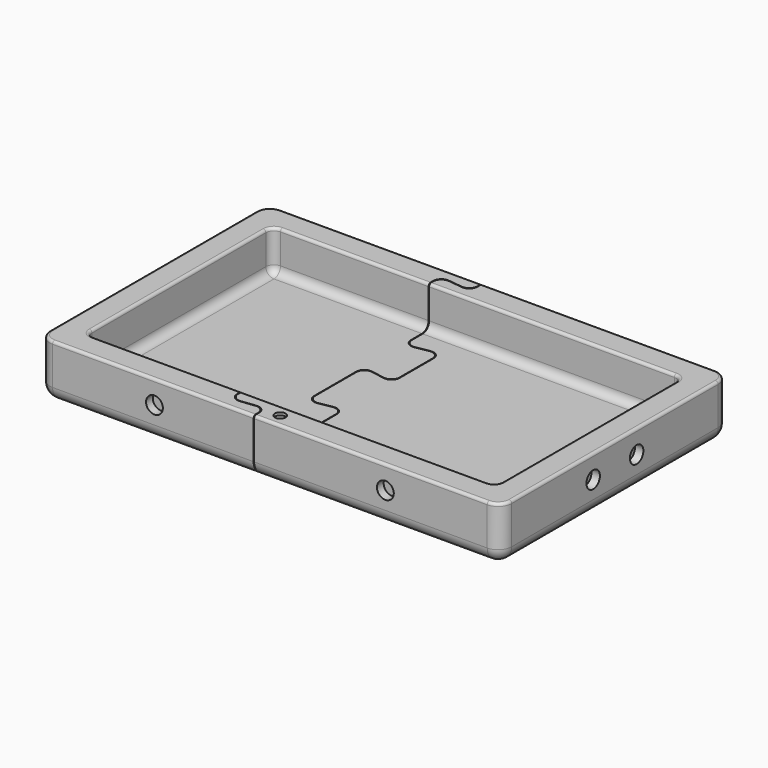
from build123d import *

# Parameters (mm, degrees)
F0_W      = 170
F0_H      = 105
F0_R      = 2
F3_DEPTH  = 20
F4_DEPTH  = 15
F5_R      = 5
F6_R      = 3
F7_R      = 1
F8_R      = 3.1
F9_DEPTH  = 3.1
F10_R     = 3.1
F11_DEPTH = 3.1
F12_R     = 3.1
F13_DEPTH = 3.1
F14_R     = 3.1
F15_DEPTH = 3.1
F16_DEPTH = 1
F17_ANGLE = 180
F19_DEPTH = 25
F20_DEPTH = 25


# Not quite as in the source:
# - a feature names something its author has since deleted; it is built from what else it names


with BuildPart() as f3:
    # F0 (on Top) → F3 (new body)
    with BuildSketch(Plane.XY):
        Rectangle(F0_W, F0_H)
        with Locations((0, -47.75)):
            Circle(F0_R, mode=Mode.SUBTRACT)
        with BuildLine():
            ThreePointArc((-75.5, 40), (-74.6213203436, 42.1213203436), (-72.5, 43))
            Line((-72.5, 43), (72.5, 43))
            ThreePointArc((72.5, 43), (74.6213203436, 42.1213203436), (75.5, 40))
            Line((75.5, 40), (75.5, -40))
            ThreePointArc((75.5, -40), (74.6213203436, -42.1213203436), (72.5, -43))
            Line((72.5, -43), (-72.5, -43))
            ThreePointArc((-72.5, -43), (-74.6213203436, -42.1213203436), (-75.5, -40))
            Line((-75.5, -40), (-75.5, 40))
        make_face(mode=Mode.SUBTRACT)
        with BuildLine():
            Line((72.5, 43), (-72.5, 43))
            ThreePointArc((-72.5, 43), (-74.6213203436, 42.1213203436), (-75.5, 40))
            Line((-75.5, 40), (-75.5, -40))
            ThreePointArc((-75.5, -40), (-74.6213203436, -42.1213203436), (-72.5, -43))
            Line((-72.5, -43), (72.5, -43))
            ThreePointArc((72.5, -43), (74.6213203436, -42.1213203436), (75.5, -40))
            Line((75.5, -40), (75.5, 40))
            ThreePointArc((75.5, 40), (74.6213203436, 42.1213203436), (72.5, 43))
        make_face()
        with Locations((0, -47.75)):
            Circle(F0_R)
    extrude(amount=F3_DEPTH)

    # F0 (on Top) → F4 (cut)
    with BuildSketch(Plane.XY):
        with BuildLine():
            Line((72.5, 43), (-72.5, 43))
            ThreePointArc((-72.5, 43), (-74.6213203436, 42.1213203436), (-75.5, 40))
            Line((-75.5, 40), (-75.5, -40))
            ThreePointArc((-75.5, -40), (-74.6213203436, -42.1213203436), (-72.5, -43))
            Line((-72.5, -43), (72.5, -43))
            ThreePointArc((72.5, -43), (74.6213203436, -42.1213203436), (75.5, -40))
            Line((75.5, -40), (75.5, 40))
            ThreePointArc((75.5, 40), (74.6213203436, 42.1213203436), (72.5, 43))
        make_face()
    extrude(amount=F4_DEPTH, mode=Mode.SUBTRACT)

    # F5
    f5_edges = [f3.edges().sort_by_distance(p)[0] for p in [
        (0, 52.5, 20),
        (-85, 0, 20),
        (0, -52.5, 20),
        (85, 0, 20),
        (85, 52.5, 10),
        (-85, 52.5, 10),
        (-85, -52.5, 10),
        (85, -52.5, 10),
    ]]
    fillet(f5_edges, radius=F5_R)

    # F6
    f6_edges = [f3.edges().sort_by_distance(p)[0] for p in [
        (0, 43, 15),
        (-74.62132, 42.12132, 15),
        (-75.5, 0, 15),
        (-74.62132, -42.12132, 15),
        (0, -43, 15),
        (74.62132, -42.12132, 15),
        (75.5, 0, 15),
        (74.62132, 42.12132, 15),
    ]]
    fillet(f6_edges, radius=F6_R)

    # F7
    f7_edges = [f3.edges().sort_by_distance(p)[0] for p in [
        (0, 52.5, 0),
        (83.535534, 51.035534, 0),
        (-83.535534, 51.035534, 0),
        (85, 0, 0),
        (-85, 0, 0),
        (83.535534, -51.035534, 0),
        (-83.535534, -51.035534, 0),
        (0, -52.5, 0),
        (0, 43, 0),
        (-74.62132, 42.12132, 0),
        (-75.5, 0, 0),
        (-74.62132, -42.12132, 0),
        (0, -43, 0),
        (74.62132, -42.12132, 0),
        (75.5, 0, 0),
        (74.62132, 42.12132, 0),
    ]]
    fillet(f7_edges, radius=F7_R)

    # F8 (on face) → F9 (cut)
    with BuildSketch(Plane.XZ.offset(52.5)):
        with Locations((42.5, 8.5)):
            Circle(F8_R)
        with Locations((-42.5, 8.5)):
            Circle(F8_R)
    extrude(amount=-F9_DEPTH, mode=Mode.SUBTRACT)

    # F10 (on face) → F11 (cut)
    with BuildSketch(Plane(origin=(0, 52.5, 0), x_dir=(-1, 0, 0), z_dir=(0, 1, 0))):
        with Locations((42.5, 8.5)):
            Circle(F10_R)
        with Locations((-42.5, 8.5)):
            Circle(F10_R)
    extrude(amount=-F11_DEPTH, mode=Mode.SUBTRACT)

    # F12 (on face) → F13 (cut)
    with BuildSketch(Plane(origin=(-85, 0, 0), x_dir=(0, -1, 0), z_dir=(-1, 0, 0))):
        with Locations((10, 8.5)):
            Circle(F12_R)
        with Locations((-10, 8.5)):
            Circle(F12_R)
    extrude(amount=-F13_DEPTH, mode=Mode.SUBTRACT)

    # F14 (on face) → F15 (cut)
    with BuildSketch(Plane.YZ.offset(85)):
        with Locations((10, 8.5)):
            Circle(F14_R)
        with Locations((-10, 8.5)):
            Circle(F14_R)
    extrude(amount=-F15_DEPTH, mode=Mode.SUBTRACT)

    # F0 (on Top) → F16 (cut)
    with BuildSketch(Plane.XY):
        with Locations((0, -47.75)):
            Circle(F0_R)
    extrude(amount=F16_DEPTH, mode=Mode.SUBTRACT)


with BuildPart() as f3_1:
    # F17: moved
    add(f3.part.rotate(Axis((0, 0, 0), (0, 1, 0)), F17_ANGLE))


with BuildPart() as f19:
    # F18 (on Top) → F19 (new body)
    with BuildSketch(Plane.XY):
        with BuildLine():
            Line((-18, -9.6620759565), (-18, 0))
            Line((-18, 0), (-18, 9.6620759565))
            ThreePointArc((-18, 9.6620759565), (-16.9283628291, 11.9602092859), (-14.479055467, 12.6164992155))
            Line((-14.479055467, 12.6164992155), (-9.520944533, 11.7422504845))
            ThreePointArc((-9.520944533, 11.7422504845), (-7.0716371709, 12.3985404142), (-6, 14.6966737436))
            Line((-6, 14.6966737436), (-6, 29.8531478456))
            ThreePointArc((-6, 29.8531478456), (-7.0716371709, 32.151281175), (-9.520944533, 32.8075711047))
            Line((-9.520944533, 32.8075711047), (-14.479055467, 31.9333223736))
            ThreePointArc((-14.479055467, 31.9333223736), (-16.9283628291, 32.5896123033), (-18, 34.8877456327))
            Line((-18, 34.8877456327), (-18, 45.1240298712))
            ThreePointArc((-18, 45.1240298712), (-16.9927715108, 47.3665422359), (-14.6474255295, 48.1032397065))
            Line((-14.6474255295, 48.1032397065), (-9.3525744705, 47.4766207667))
            ThreePointArc((-9.3525744705, 47.4766207667), (-7.0072284892, 48.2133182373), (-6, 50.455830602))
            Line((-6, 50.455830602), (-6, 69.1191965569))
            Line((-6, 69.1191965569), (-107.2437387941, 69.1191965569))
            Line((-107.2437387941, 69.1191965569), (-107.2437387941, 0))
            Line((-107.2437387941, 0), (-107.2437387941, -69.1191965569))
            Line((-107.2437387941, -69.1191965569), (-6, -69.1191965569))
            Line((-6, -69.1191965569), (-6, -50.455830602))
            ThreePointArc((-6, -50.455830602), (-7.0072284892, -48.2133182373), (-9.3525744705, -47.4766207667))
            Line((-9.3525744705, -47.4766207667), (-14.6474255295, -48.1032397065))
            ThreePointArc((-14.6474255295, -48.1032397065), (-16.9927715108, -47.3665422359), (-18, -45.1240298712))
            Line((-18, -45.1240298712), (-18, -34.8877456327))
            ThreePointArc((-18, -34.8877456327), (-16.9283628291, -32.5896123033), (-14.479055467, -31.9333223736))
            Line((-14.479055467, -31.9333223736), (-9.520944533, -32.8075711047))
            ThreePointArc((-9.520944533, -32.8075711047), (-7.0716371709, -32.151281175), (-6, -29.8531478456))
            Line((-6, -29.8531478456), (-6, -14.6966737436))
            ThreePointArc((-6, -14.6966737436), (-7.0716371709, -12.3985404142), (-9.520944533, -11.7422504845))
            Line((-9.520944533, -11.7422504845), (-14.479055467, -12.6164992155))
            ThreePointArc((-14.479055467, -12.6164992155), (-16.9283628291, -11.9602092859), (-18, -9.6620759565))
        make_face()
    extrude(amount=-F19_DEPTH)


with BuildPart() as f20:
    # F18 (on Top) → F20 (new body)
    with BuildSketch(Plane.XY):
        with BuildLine():
            Line((108.1050901483, 69.1191965569), (-5.8, 69.1191965569))
            Line((-5.8, 69.1191965569), (-5.8, 50.2307659268))
            ThreePointArc((-5.8, 50.2307659268), (-6.8072284892, 47.9882535621), (-9.1525744705, 47.2515560915))
            Line((-9.1525744705, 47.2515560915), (-14.4474255295, 47.8781750312))
            ThreePointArc((-14.4474255295, 47.8781750312), (-16.7927715108, 47.1414775606), (-17.8, 44.8989651959))
            Line((-17.8, 44.8989651959), (-17.8, 35.1260963512))
            ThreePointArc((-17.8, 35.1260963512), (-16.7283628291, 32.8279630218), (-14.279055467, 32.1716730922))
            Line((-14.279055467, 32.1716730922), (-9.320944533, 33.0459218232))
            ThreePointArc((-9.320944533, 33.0459218232), (-6.8716371709, 32.3896318935), (-5.8, 30.0914985641))
            Line((-5.8, 30.0914985641), (-5.8, 14.4583230251))
            ThreePointArc((-5.8, 14.4583230251), (-6.8716371709, 12.1601896957), (-9.320944533, 11.503899766))
            Line((-9.320944533, 11.503899766), (-14.279055467, 12.378148497))
            ThreePointArc((-14.279055467, 12.378148497), (-16.7283628291, 11.7218585673), (-17.8, 9.423725238))
            Line((-17.8, 9.423725238), (-17.8, 0))
            Line((-17.8, 0), (-17.8, -9.423725238))
            ThreePointArc((-17.8, -9.423725238), (-16.7283628291, -11.7218585673), (-14.279055467, -12.378148497))
            Line((-14.279055467, -12.378148497), (-9.320944533, -11.503899766))
            ThreePointArc((-9.320944533, -11.503899766), (-6.8716371709, -12.1601896957), (-5.8, -14.4583230251))
            Line((-5.8, -14.4583230251), (-5.8, -30.0914985641))
            ThreePointArc((-5.8, -30.0914985641), (-6.8716371709, -32.3896318935), (-9.320944533, -33.0459218232))
            Line((-9.320944533, -33.0459218232), (-14.279055467, -32.1716730922))
            ThreePointArc((-14.279055467, -32.1716730922), (-16.7283628291, -32.8279630218), (-17.8, -35.1260963512))
            Line((-17.8, -35.1260963512), (-17.8, -44.8989651959))
            ThreePointArc((-17.8, -44.8989651959), (-16.7927715108, -47.1414775606), (-14.4474255295, -47.8781750312))
            Line((-14.4474255295, -47.8781750312), (-9.1525744705, -47.2515560915))
            ThreePointArc((-9.1525744705, -47.2515560915), (-6.8072284892, -47.9882535621), (-5.8, -50.2307659268))
            Line((-5.8, -50.2307659268), (-5.8, -69.1191965569))
            Line((-5.8, -69.1191965569), (108.1050901483, -69.1191965569))
            Line((108.1050901483, -69.1191965569), (108.1050901483, 69.1191965569))
        make_face()
    extrude(amount=-F20_DEPTH)


with BuildPart() as f21_1:
    # F21: copy of F3
    add(f3_1.part)


with BuildPart() as f3_2:
    add(f3_1.part)

    # F22: intersect F19
    add(f19.part, mode=Mode.INTERSECT)


with BuildPart() as f20_1:
    add(f20.part)

    # F23: intersect F21_1
    add(f21_1.part, mode=Mode.INTERSECT)


solid = Compound([f3_2.part, f20_1.part])
